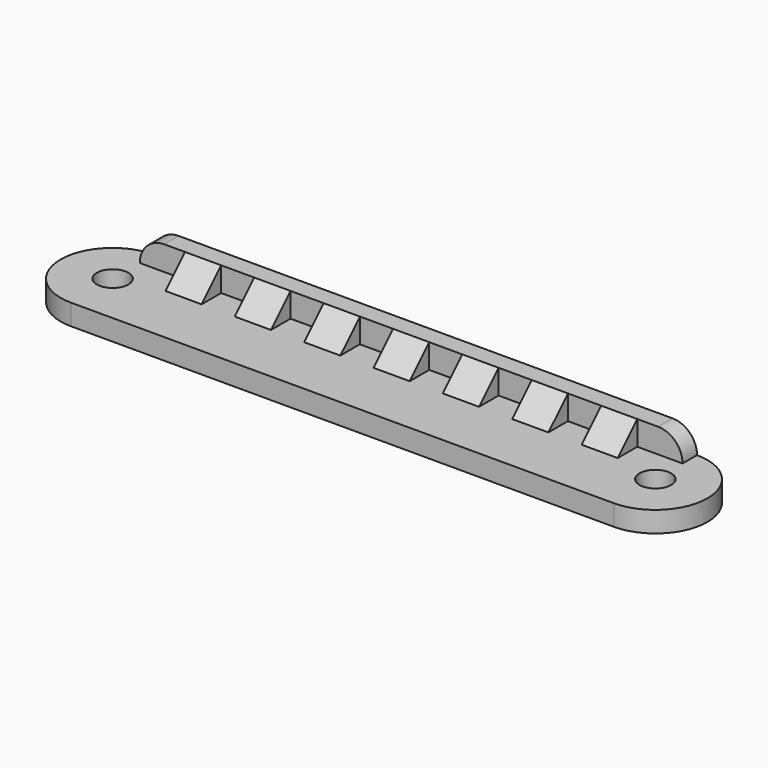
from build123d import *

# Parameters (mm, degrees)
F0_R     = 1.75
F1_DEPTH = 2.3
F0_W     = 60
F0_H     = 2
F2_DEPTH = 5
F3_W     = 4
F3_H     = 2.7
F4_DEPTH = 2.7
F5_SIZE  = 2.69999
F6_R     = 2.69999


# Not quite as in the source:
# - a fillet or chamfer is up to 0.001 mm smaller than in the source, because OpenCascade refuses the exact size


with BuildPart() as f1:
    # F0 (on Top) → F1 (new body)
    with BuildSketch(Plane.XY):
        with BuildLine():
            Line((-30, 3.75), (-30, 5.75))
            ThreePointArc((-30, 5.75), (-35.75, 0), (-30, -5.75))
            Line((-30, -5.75), (30, -5.75))
            ThreePointArc((30, -5.75), (35.75, 0), (30, 5.75))
            Line((30, 5.75), (30, 3.75))
            Line((30, 3.75), (-30, 3.75))
        make_face()
        with Locations((-30, 0)):
            Circle(F0_R, mode=Mode.SUBTRACT)
        with Locations((30, 0)):
            Circle(F0_R, mode=Mode.SUBTRACT)
    extrude(amount=F1_DEPTH)

    # F0 (on Top) → F2 (join)
    with BuildSketch(Plane.XY):
        with Locations((0, 4.75)):
            Rectangle(F0_W, F0_H)
    extrude(amount=F2_DEPTH)

    # F3 (on face) → F4 (join, through all)
    with BuildSketch(Plane.XY.offset(2.3)):
        with Locations((-23, 2.4)):
            Rectangle(F3_W, F3_H)
        with Locations((-15.3333333333, 2.4)):
            Rectangle(F3_W, F3_H)
        with Locations((-7.6666666667, 2.4)):
            Rectangle(F3_W, F3_H)
        with Locations((0, 2.4)):
            Rectangle(F3_W, F3_H)
        with Locations((7.6666666667, 2.4)):
            Rectangle(F3_W, F3_H)
        with Locations((15.3333333333, 2.4)):
            Rectangle(F3_W, F3_H)
        with Locations((23, 2.4)):
            Rectangle(F3_W, F3_H)
    extrude(amount=F4_DEPTH)

    # F5 (size 2.7 in the source; OpenCascade refuses exactly that, so slightly less here)
    f5_edges = [f1.edges().sort_by_distance(p)[0] for p in [
        (-23, 1.05, 5),
        (-15.333333, 1.05, 5),
        (-7.666667, 1.05, 5),
        (0, 1.05, 5),
        (7.666667, 1.05, 5),
        (15.333333, 1.05, 5),
        (23, 1.05, 5),
    ]]
    chamfer(f5_edges, length=F5_SIZE)

    # F6 (radius 2.7 in the source; OpenCascade refuses exactly that, so slightly less here)
    f6_edges = [f1.edges().sort_by_distance(p)[0] for p in [
        (30, 4.75, 5),
        (-30, 4.75, 5),
    ]]
    fillet(f6_edges, radius=F6_R)


solid = f1.part
